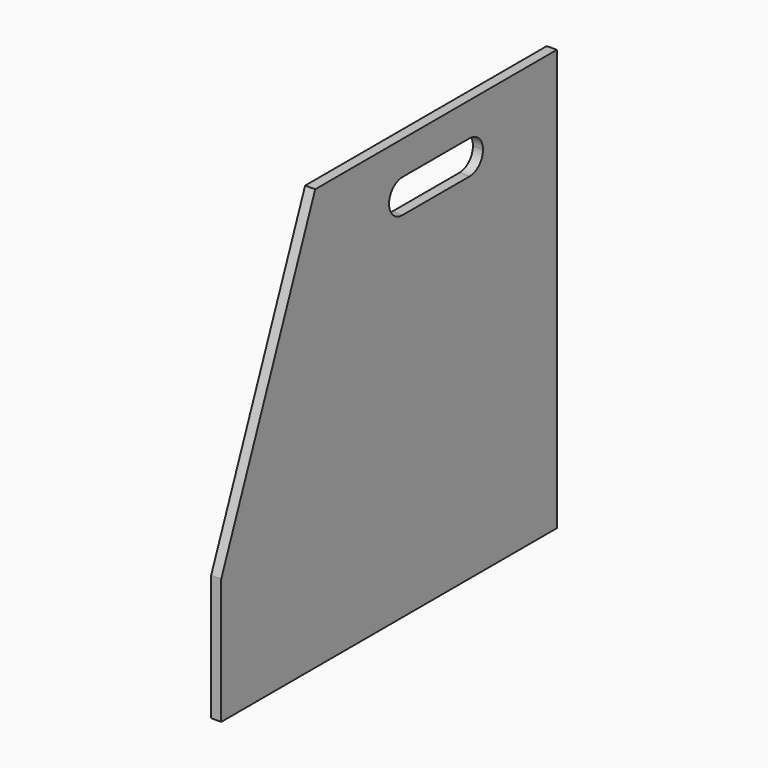
from build123d import *

# Parameters (mm, degrees)
F0_W      = 500
F0_H      = 500
F1_DEPTH  = 12
F2_W      = 500
F2_H      = 50
F3_DEPTH  = 6
F6_DEPTH  = 6
F14_DEPTH = 6
F15_R     = 19.99999
F19_DEPTH = 6
F22_DEPTH = 12
F25_DEPTH = 6
F27_W     = 12
F27_H     = 320
F28_DEPTH = 44
F31_W     = 196
F31_H     = 12
F32_DEPTH = 44
F37_DEPTH = 3
F43_DEPTH = 12


# Not quite as in the source:
# - a fillet or chamfer is up to 0.001 mm smaller than in the source, because OpenCascade refuses the exact size


with BuildPart() as f1:
    # F0 (on Top) → F1 (new body)
    with BuildSketch(Plane.XY):
        Rectangle(F0_W, F0_H)
    extrude(amount=F1_DEPTH)


with BuildPart() as f3:
    # F2 (on Right) → F3 (new body, symmetric)
    with BuildSketch(Plane.YZ):
        Rectangle(F2_W, F2_H)
    extrude(amount=F3_DEPTH, both=True)


with BuildPart() as f3_1:
    # F4: moved
    add(f3.part.moved(Location((0, 0, -25))))


with BuildPart() as f6:
    # F5 (on Front) → F6 (new body, symmetric)
    with BuildSketch(Plane.XZ):
        Polygon((-250, -25), (250, -25), (250, 25), (6, 25), (6, 0), (-6, 0), (-6, 25), (-250, 25), align=None)
    extrude(amount=F6_DEPTH, both=True)


with BuildPart() as f6_1:
    # F7: moved
    add(f6.part.moved(Location((0, 80, -25))))


with BuildPart() as f8_1:
    # F8: copy of F6
    add(f6_1.part)


with BuildPart() as f3_2:
    add(f3_1.part)

    # F10: cut F6
    add(f6_1.part, mode=Mode.SUBTRACT)


with BuildPart() as f11_1:
    # F11: copy of F6
    add(f6_1.part.moved(Location((0, 164, 0))))


with BuildPart() as f3_3:
    add(f3_2.part)

    # F12: cut F11_1
    add(f11_1.part, mode=Mode.SUBTRACT)


with BuildPart() as f14:
    # F13 (on Right) → F14 (new body, symmetric)
    with BuildSketch(Plane.YZ):
        Polygon((250, -50), (250, 0), (250, 452), (70, 452), (-110, 452), (-250, 100), (-250, -50), align=None)
        Polygon((0, 412), (70, 412), (140, 412), (140, 372), (0, 372), align=None, mode=Mode.SUBTRACT)
    extrude(amount=F14_DEPTH, both=True)

    # F15 (radius 20 in the source; OpenCascade refuses exactly that, so slightly less here)
    f15_edges = [f14.edges().sort_by_distance(p)[0] for p in [
        (0, 140, 372),
        (0, 140, 412),
        (0, 0, 412),
        (0, 0, 372),
    ]]
    fillet(f15_edges, radius=F15_R)


with BuildPart() as f14_1:
    # F16: moved
    add(f14.part.moved(Location((-256, 0, 0))))


with BuildPart() as f17_1:
    # F17: copy of F14
    add(f14_1.part.moved(Location((512, 0, 0))))


with BuildPart() as f19:
    # F18 (on Front) → F19 (new body, symmetric)
    with BuildSketch(Plane.XZ):
        Polygon((-262, 452), (-262, 0), (-262, -50), (262, -50), (262, 452), align=None)
    extrude(amount=F19_DEPTH, both=True)


with BuildPart() as f19_1:
    # F20: moved
    add(f19.part.moved(Location((0, 256, 0))))


with BuildPart() as f22:
    # F21 (on face) → F22 (new body)
    with BuildSketch(Plane.XY.offset(12)):
        Polygon((262, 262), (0, 262), (-262, 262), (-262, -110), (262, -110), align=None)
    extrude(amount=F22_DEPTH)


with BuildPart() as f22_1:
    # F23: moved
    add(f22.part.moved(Location((0, 0, 440))))


with BuildPart() as f25:
    # F24 (on Front) → F25 (new body, symmetric)
    with BuildSketch(Plane.XZ):
        Polygon((-250, 12), (0, 12), (250, 12), (250, 100), (-250, 100), align=None)
    extrude(amount=F25_DEPTH, both=True)


with BuildPart() as f25_1:
    # F26: moved
    add(f25.part.moved(Location((0, -244, 0))))


with BuildPart() as f28:
    # F27 (on Top) → F28 (new body)
    with BuildSketch(Plane.XY):
        with Locations((-24, -90)):
            Rectangle(F27_W, F27_H)
    extrude(amount=F28_DEPTH)


with BuildPart() as f28_1:
    # F29: moved
    add(f28.part.moved(Location((0, 0, -48))))


with BuildPart() as f30_1:
    # F30: copy of F28
    add(f28_1.part.moved(Location((-208, 0, 0))))


with BuildPart() as f32:
    # F31 (on Top) → F32 (new body)
    with BuildSketch(Plane.XY):
        with Locations((-128, -244)):
            Rectangle(F31_W, F31_H)
    extrude(amount=-F32_DEPTH)


with BuildPart() as f32_1:
    # F33: moved
    add(f32.part.moved(Location((0, 0, -4))))


with BuildPart() as f34_1:
    # F34: copy of F32
    add(f32_1.part.moved(Location((0, 308, 0))))


with BuildPart() as f35_1:
    # F35: copy of F32
    add(f32_1.part.moved(Location((256, 0, 0))))


with BuildPart() as f35_2:
    # F35: copy of F30_1
    add(f30_1.part.moved(Location((256, 0, 0))))


with BuildPart() as f35_3:
    # F35: copy of F28
    add(f28_1.part.moved(Location((256, 0, 0))))


with BuildPart() as f35_4:
    # F35: copy of F34_1
    add(f34_1.part.moved(Location((256, 0, 0))))


with BuildPart() as f37:
    # F36 (on Top) → F37 (new body)
    with BuildSketch(Plane.XY):
        Polygon((-24, -244), (-24, 0), (-24, 64), (-232, 64), (-232, -244), align=None)
    extrude(amount=F37_DEPTH)


with BuildPart() as f37_1:
    # F38: moved
    add(f37.part.moved(Location((0, 0, -44))))


with BuildPart() as f39_1:
    # F39: copy of F37
    add(f37_1.part.moved(Location((256, 0, 0))))


with BuildPart() as f30_1_1:
    add(f30_1.part)

    # F40: cut F37
    add(f37_1.part, mode=Mode.SUBTRACT)


with BuildPart() as f32_2:
    add(f32_1.part)

    # F40: cut F37
    add(f37_1.part, mode=Mode.SUBTRACT)


with BuildPart() as f28_2:
    add(f28_1.part)

    # F40: cut F37
    add(f37_1.part, mode=Mode.SUBTRACT)


with BuildPart() as f34_1_1:
    add(f34_1.part)

    # F40: cut F37
    add(f37_1.part, mode=Mode.SUBTRACT)


with BuildPart() as f35_1_1:
    add(f35_1.part)

    # F41: cut F39_1
    add(f39_1.part, mode=Mode.SUBTRACT)


with BuildPart() as f35_3_1:
    add(f35_3.part)

    # F41: cut F39_1
    add(f39_1.part, mode=Mode.SUBTRACT)


with BuildPart() as f35_4_1:
    add(f35_4.part)

    # F41: cut F39_1
    add(f39_1.part, mode=Mode.SUBTRACT)


with BuildPart() as f35_2_1:
    add(f35_2.part)

    # F41: cut F39_1
    add(f39_1.part, mode=Mode.SUBTRACT)


with BuildPart() as f43:
    # F42 (on Front) → F43 (new body)
    with BuildSketch(Plane.XZ):
        Polygon((0, 12), (0, 0), (0, -50), (262, -50), (262, 12), align=None)
    extrude(amount=F43_DEPTH)


with BuildPart() as f43_1:
    # F44: moved
    add(f43.part.moved(Location((0, -250, 0))))


with BuildPart() as f45_1:
    # F45: copy of F43
    add(f43_1.part.moved(Location((-262, 0, 0))))


solid = f14_1.part
